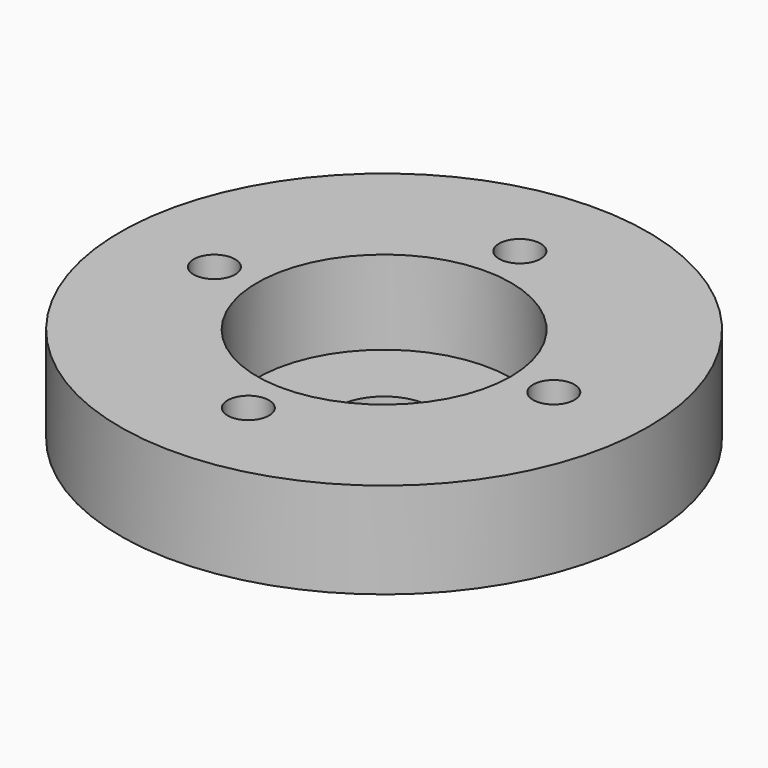
from build123d import *

# Parameters (mm, degrees)
F0_W           = 92.075
F0_H           = 12.7
F1_DEPTH       = 46.0375
F2_R           = 16.8275
F3_DEPTH       = 11.1125
F4_D           = 5.5
F5_R           = 35
F5_R_2         = 16.8275
F6_DEPTH       = 25.4
F7_D           = 12.7
F7_CBORE_D     = 12.7
F7_CBORE_DEPTH = 6.35


# Not quite as in the source:
# - a length typed as a fraction of an inch, garbled in the dataset ("3 / 203.2 mm" for 3/8 in), is restored


with BuildPart() as f1:
    # F0 (on Front) → F1 (new body, symmetric)
    with BuildSketch(Plane.XZ):
        with Locations((7.9375, 6.35)):
            Rectangle(F0_W, F0_H)
    extrude(amount=F1_DEPTH, both=True)

    # F2 (on face) → F3 (cut)
    with BuildSketch(Plane.XY.offset(12.7)):
        Circle(F2_R)
    extrude(amount=-F3_DEPTH, mode=Mode.SUBTRACT)

    # F4 (through all)
    with Locations(Plane.XY.offset(12.7)):
        with Locations((0, 22.5), (22.5, 0), (0, -22.5), (-22.5, 0)):
            Hole(F4_D / 2)

    # F5 (on face) → F6 (intersect)
    with BuildSketch(Plane.XY.offset(12.7)):
        Circle(F5_R)
        Circle(F5_R_2, mode=Mode.SUBTRACT)
        Circle(F5_R_2)
    extrude(amount=-F6_DEPTH, mode=Mode.INTERSECT)

    # F7 (through all)
    with Locations(Plane.XY.offset(12.7)):
        with Locations((0, 0)):
            CounterBoreHole(F7_D / 2, F7_CBORE_D / 2, F7_CBORE_DEPTH)


solid = f1.part
